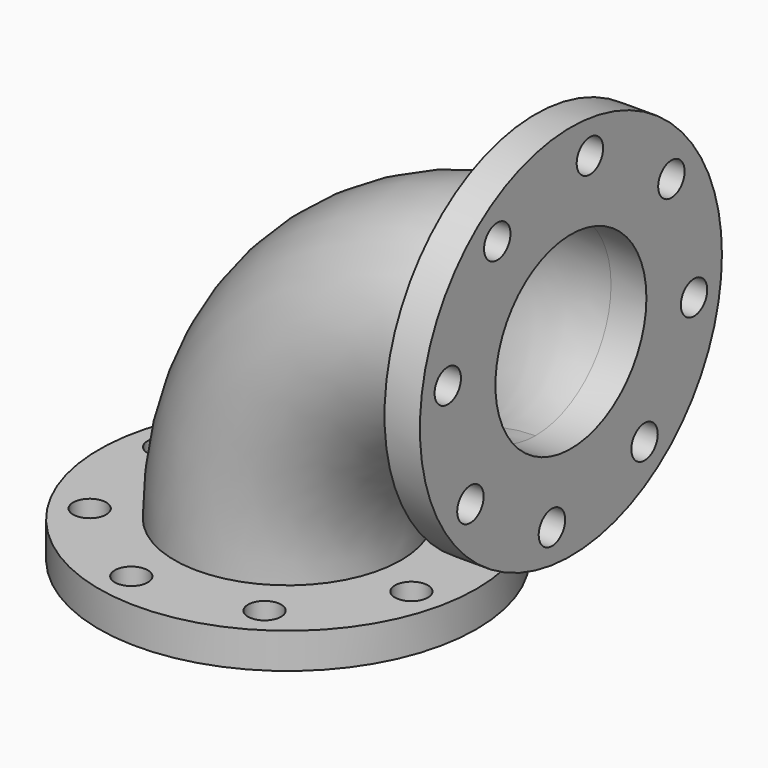
from build123d import *

# Parameters (mm, degrees)
F2_R     = 127
F2_R_2   = 11.1125
F2_R_3   = 63.5
F3_DEPTH = 23.8125
F5_ANGLE = 90
F0_R     = 127
F0_R_2   = 11.1125
F0_R_3   = 63.5
F6_DEPTH = 23.8252


with BuildPart() as f3:
    # F2 (on offset) → F3 (new body)
    with BuildSketch(Plane.YZ.offset(190.5)):
        with Locations((0, 190.9857690334)):
            Circle(F2_R)
        with Locations((-15.9666395956, 87.4344916631)):
            Circle(F2_R_2, mode=Mode.SUBTRACT)
        with Locations((-84.5119295599, 129.0540777352)):
            Circle(F2_R_2, mode=Mode.SUBTRACT)
        with Locations((61.9316912983, 106.4738394735)):
            Circle(F2_R_2, mode=Mode.SUBTRACT)
        with Locations((103.5512773703, 175.0191294378)):
            Circle(F2_R_2, mode=Mode.SUBTRACT)
        with Locations((-103.5512773703, 206.952408629)):
            Circle(F2_R_2, mode=Mode.SUBTRACT)
        with Locations((-61.9316912983, 275.4976985933)):
            Circle(F2_R_2, mode=Mode.SUBTRACT)
        with Locations((0, 190.9857690334)):
            Circle(F2_R_3, mode=Mode.SUBTRACT)
        with Locations((84.5119295599, 252.9174603317)):
            Circle(F2_R_2, mode=Mode.SUBTRACT)
        with Locations((15.9666395956, 294.5370464037)):
            Circle(F2_R_2, mode=Mode.SUBTRACT)
    extrude(amount=-F3_DEPTH)

    # F4 (on face) → F5 (revolve)
    with BuildSketch(Plane(origin=(166.6875, 0, 0), x_dir=(0, -1, 0), z_dir=(-1, 0, 0))):
        with BuildLine():
            ThreePointArc((76.2, 190.9857690334), (-53.8815367264, 244.8673057598), (0, 114.7857690334))
            ThreePointArc((0, 114.7857690334), (53.8815367264, 137.104232307), (76.2, 190.9857690334))
        make_face()
        with BuildLine():
            ThreePointArc((0, 127.4857690334), (-44.9012806053, 235.8870496388), (63.5, 190.9857690334))
            ThreePointArc((63.5, 190.9857690334), (44.9012806053, 146.0844884281), (0, 127.4857690334))
        make_face(mode=Mode.SUBTRACT)
    revolve(axis=Axis((166.6875, -174.7182756662, 24.2982690334), (0, -1, 0)), revolution_arc=F5_ANGLE)


with BuildPart() as f6:
    # F0 (on Top) → F6 (new body)
    with BuildSketch(Plane.XY):
        Circle(F0_R)
        with Locations((-23.6012563885, -102.0822282373)):
            Circle(F0_R_2, mode=Mode.SUBTRACT)
        with Locations((-88.871644262, -55.4944273884)):
            Circle(F0_R_2, mode=Mode.SUBTRACT)
        with Locations((55.4944273884, -88.871644262)):
            Circle(F0_R_2, mode=Mode.SUBTRACT)
        with Locations((102.0822282373, -23.6012563885)):
            Circle(F0_R_2, mode=Mode.SUBTRACT)
        with Locations((-102.0822282373, 23.6012563885)):
            Circle(F0_R_2, mode=Mode.SUBTRACT)
        with Locations((-55.4944273884, 88.871644262)):
            Circle(F0_R_2, mode=Mode.SUBTRACT)
        Circle(F0_R_3, mode=Mode.SUBTRACT)
        with Locations((88.871644262, 55.4944273884)):
            Circle(F0_R_2, mode=Mode.SUBTRACT)
        with Locations((23.6012563885, 102.0822282373)):
            Circle(F0_R_2, mode=Mode.SUBTRACT)
    extrude(amount=F6_DEPTH)


solid = Compound([f3.part, f6.part])
